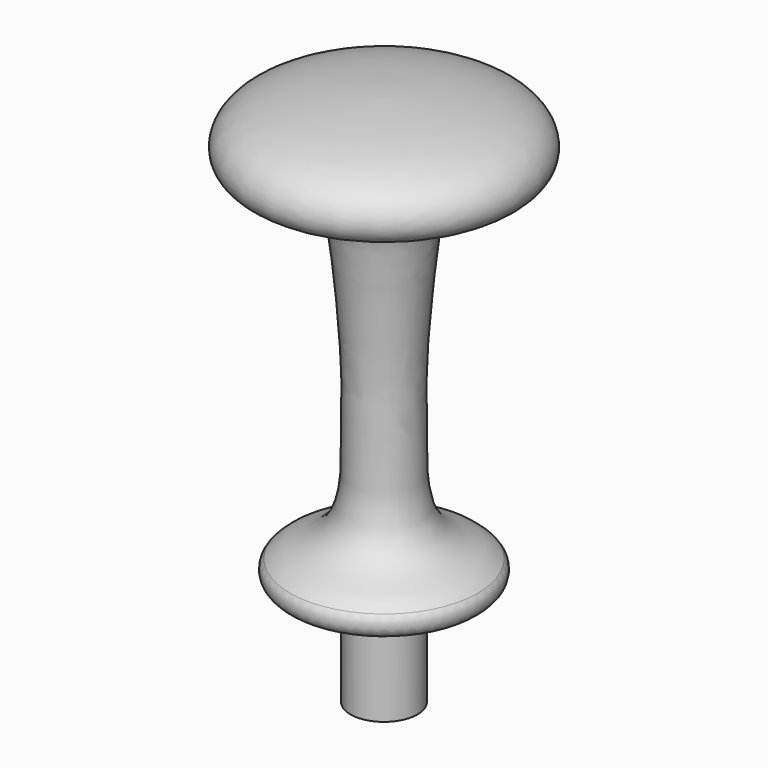
from build123d import *

# Parameters (mm, degrees)
F3_R     = 2.54
F4_R     = 1.5875
F5_DEPTH = 19.05


# Not quite as in the source:
# - a fillet or chamfer that OpenCascade refuses, or shapes differently, is made with other operations: its cross-section is extruded or revolved along the edge and cut away or added


with BuildPart() as f1:
    # F0 (on Front) → F1 (revolve)
    with BuildSketch(Plane.XZ):
        with BuildLine():
            Line((-6.35, 0), (0, 0))
            Line((0, 0), (0, 101.6))
            add(Edge.make_bspline(
                [(-19.05, 22.225), (-17.8017115835, 24.3033621055), (-15.1804667376, 25.8563995583), (-5.8587234356, 29.5839922823), (-6.522784631, 46.7742284873), (-6.1049370074, 54.205364509), (-7.3072341458, 70.5428303924), (-8.1967484803, 77.1861874567), (-9.183875058, 86.588833183), (-18.6288397232, 87.0163776627), (-26.8817407745, 89.5937070669), (-25.1675530586, 99.3024571105), (-6.0102460072, 101.5650457629), (-1.9329084316, 101.5911921859), (0, 101.6)],
                knots=[0, 0, 0, 0, 0.0641397989, 0.143349521, 0.2508366946, 0.3318774546, 0.4397884556, 0.5150027416, 0.5905352132, 0.6705112049, 0.7454850538, 0.8147944501, 0.9308806068, 1, 1, 1, 1], degree=3))
            Line((-19.05, 22.225), (-19.05, 19.05))
            Line((-19.05, 19.05), (-6.35, 19.05))
            Line((-6.35, 19.05), (-6.35, 0))
        make_face()
    revolve(axis=Axis((0, 0, 50.8), (0, 0, 1)))

    # F2: fillet of radius 5.08 on 1 edges, made by hand

    # F2_s1 → F2_t2 (revolve, cut)
    with BuildSketch(Plane.XZ):
        with BuildLine():
            ThreePointArc((-19.05, 22.225), (-17.1805202921, 19.9178865162), (-14.3407139607, 19.05))
            Line((-14.3407139607, 19.05), (-19.05, 19.05))
            Line((-19.05, 19.05), (-19.05, 22.225))
        make_face()
    revolve(axis=Axis((0, 0, 19.05), (0, 0, 1)), mode=Mode.SUBTRACT)

    # F3
    f3_edges = [f1.edges().sort_by_distance(p)[0] for p in [
        (19.05, 0, 22.225),
    ]]
    fillet(f3_edges, radius=F3_R)

    # F4 (on face) → F5 (cut)
    with BuildSketch(Plane(origin=(0, 0, 0), x_dir=(1, 0, 0), z_dir=(0, 0, -1))):
        Circle(F4_R)
    extrude(amount=-F5_DEPTH, mode=Mode.SUBTRACT)


solid = f1.part
